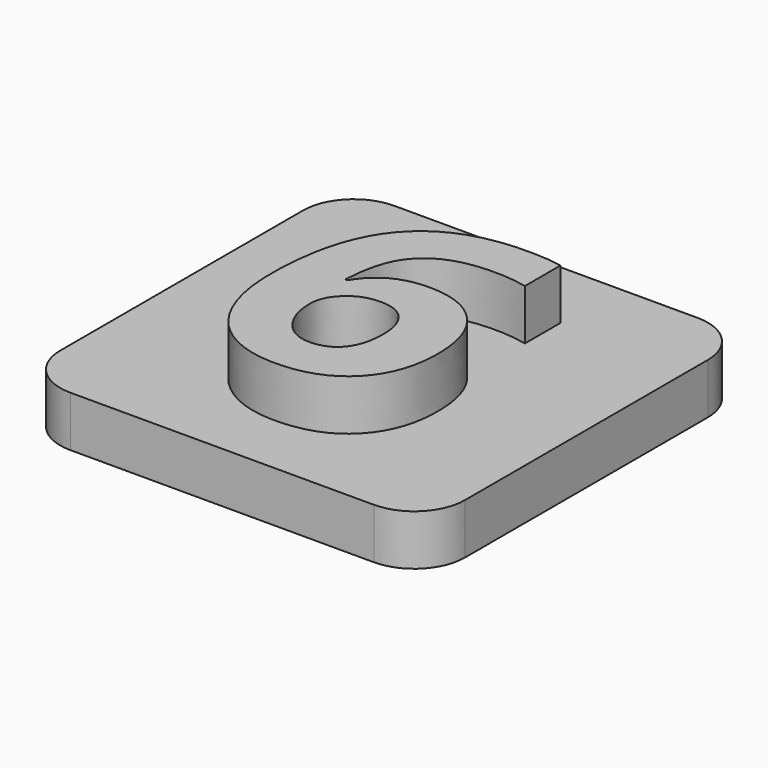
from build123d import *

# Parameters (mm, degrees)
F1_DEPTH     = 6.35
F2_TEXT_SIZE = 46.4634141988
F3_DEPTH     = 6.35


# Not quite as in the source:
# - Text() gives the source's letters only with a copy of the font that has no kerning and outlines rounded to 1/6400 em; it was checked with that copy


with BuildPart() as f1:
    # F0 (on Top) → F1 (new body)
    with BuildSketch(Plane.XY):
        with BuildLine():
            Line((-16.2467067897, 64.1814634755), (-54.3467067897, 64.1814634755))
            ThreePointArc((-54.3467067897, 64.1814634755), (-58.8368348503, 62.3215915361), (-60.6967067897, 57.8314634755))
            Line((-60.6967067897, 57.8314634755), (-60.6967067897, 19.7314634755))
            ThreePointArc((-60.6967067897, 19.7314634755), (-58.8368348503, 15.241335415), (-54.3467067897, 13.3814634755))
            Line((-54.3467067897, 13.3814634755), (-16.2467067897, 13.3814634755))
            ThreePointArc((-16.2467067897, 13.3814634755), (-11.7565787292, 15.241335415), (-9.8967067897, 19.7314634755))
            Line((-9.8967067897, 19.7314634755), (-9.8967067897, 57.8314634755))
            ThreePointArc((-9.8967067897, 57.8314634755), (-11.7565787292, 62.3215915361), (-16.2467067897, 64.1814634755))
        make_face()
    extrude(amount=F1_DEPTH)

    # F2 (on face) → F3 (join)
    with BuildSketch(Plane.XY.offset(6.35)):
        with Locations((-48.7865842879, 21.7448771)):
            Text('6', F2_TEXT_SIZE, font='Open Sans', font_style=FontStyle.BOLD, text_align=(TextAlign.LEFT, TextAlign.BOTTOM))
    extrude(amount=F3_DEPTH)


solid = f1.part
